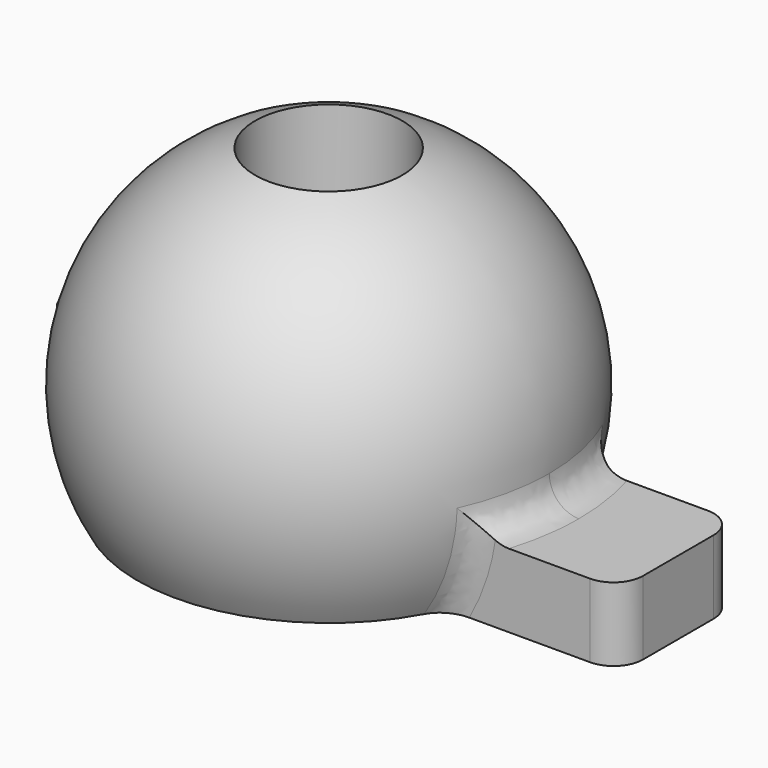
from build123d import *

# Parameters (mm, degrees)
F2_R     = 12.7
F3_DEPTH = 76.2
F5_DEPTH = 12.7
F6_R     = 5.08


# Not quite as in the source:
# - two fillets or chamfers of one size are made in one step


with BuildPart() as f1:
    # F0 (on Front) → F1 (revolve)
    with BuildSketch(Plane.XZ):
        with BuildLine():
            Line((0, -19.05), (32.9955678842, -19.05))
            ThreePointArc((32.9955678842, -19.05), (32.9955678842, 19.05), (0, 38.1))
            Line((0, 38.1), (0, -19.05))
        make_face()
    revolve(axis=Axis((0, 0, 9.525), (0, 0, 1)))

    # F2 (on Top) → F3 (cut, symmetric)
    with BuildSketch(Plane.XY):
        Circle(F2_R)
    extrude(amount=F3_DEPTH, both=True, mode=Mode.SUBTRACT)

    # F4 (on face) → F5 (join)
    with BuildSketch(Plane(origin=(0, 0, -19.05), x_dir=(1, 0, 0), z_dir=(0, 0, -1))):
        with BuildLine():
            Line((30.453530173, -12.7), (60.325, -12.7))
            Line((60.325, -12.7), (60.325, 12.7))
            Line((60.325, 12.7), (30.453530173, 12.7))
            ThreePointArc((30.453530173, 12.7), (32.3538175656, 6.4759546733), (32.9955678842, 0))
            ThreePointArc((32.9955678842, 0), (32.3538175656, -6.4759546733), (30.453530173, -12.7))
        make_face()
        with BuildLine():
            Line((4.87e-08, -12.7), (30.453530173, -12.7))
            ThreePointArc((30.453530173, -12.7), (32.3538175656, -6.4759546733), (32.9955678842, 0))
            ThreePointArc((32.9955678842, 0), (32.3538175656, 6.4759546733), (30.453530173, 12.7))
            Line((30.453530173, 12.7), (-1.16e-08, 12.7))
            ThreePointArc((-1.16e-08, 12.7), (8.980256117, 8.9802561252), (12.7, 0))
            ThreePointArc((12.7, 0), (8.9802561383, -8.9802561039), (4.87e-08, -12.7))
        make_face()
        with BuildLine():
            Line((-30.453530173, -12.7), (4.87e-08, -12.7))
            ThreePointArc((4.87e-08, -12.7), (-12.7, -3.01e-08), (-1.16e-08, 12.7))
            Line((-1.16e-08, 12.7), (-30.453530173, 12.7))
            ThreePointArc((-30.453530173, 12.7), (-32.9955678842, 0), (-30.453530173, -12.7))
        make_face()
        with BuildLine():
            Line((-60.325, -12.7), (-30.453530173, -12.7))
            ThreePointArc((-30.453530173, -12.7), (-32.9955678842, 0), (-30.453530173, 12.7))
            Line((-30.453530173, 12.7), (-60.325, -12.7))
        make_face()
    extrude(amount=-F5_DEPTH)

    # F6
    f6_edges = [f1.edges().sort_by_distance(p)[0] for p in [
        (33.511538, -12.7, -12.934328),
        (37.010025, -6.445581, -6.35),
        (37.010025, 6.445581, -6.35),
        (-60.325, 12.7, -12.7),
        (-33.511538, 12.7, -12.934328),
        (33.511538, 12.7, -12.934328),
        (60.325, -12.7, -12.7),
        (60.325, 12.7, -12.7),
        (-37.460663, 2.825994, -6.35),
        (-34.437045, -9.312779, -13.378045),
    ]]
    fillet(f6_edges, radius=F6_R)


solid = f1.part
